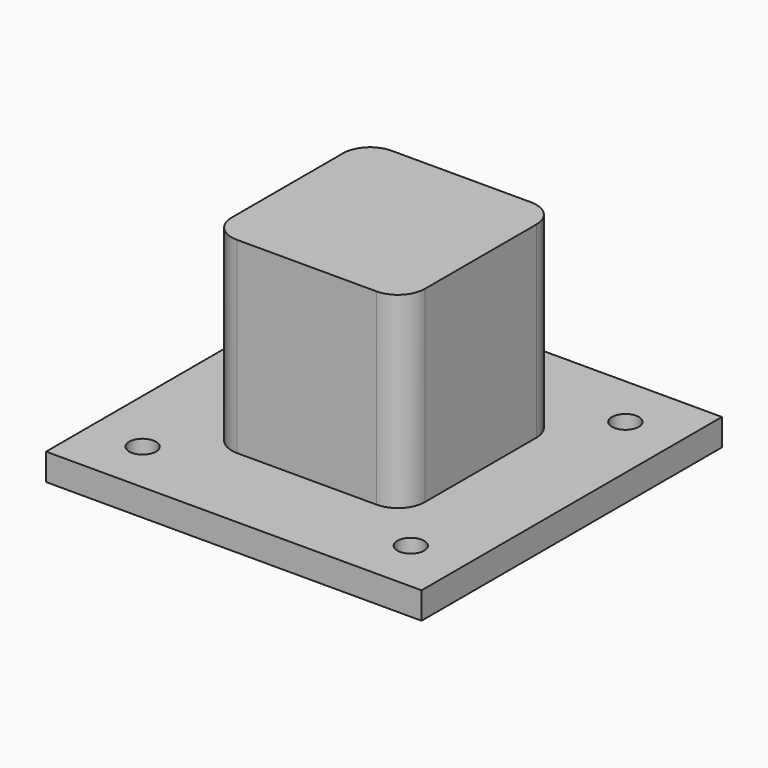
from build123d import *

# Parameters (mm, degrees)
F0_W     = 70
F0_H     = 70
F1_DEPTH = 5
F2_D     = 5
F3_W     = 36
F3_H     = 36
F4_DEPTH = 35
F5_R     = 5


# Not quite as in the source:
# - a feature names something its author has since deleted; it is built from what else it names


with BuildPart() as f1:
    # F0 (on Top) → F1 (new body)
    with BuildSketch(Plane.XY):
        Rectangle(F0_W, F0_H)
    extrude(amount=F1_DEPTH)

    # F2 (through all)
    with Locations(Plane(origin=(0, 0, 0), x_dir=(1, 0, 0), z_dir=(0, 0, -1))):
        with Locations((-25, -25), (25, -25), (25, 25), (-25, 25)):
            Hole(F2_D / 2)

    # F3 (on face) → F4 (join)
    with BuildSketch(Plane.XY.offset(5)):
        Rectangle(F3_W, F3_H)
    extrude(amount=F4_DEPTH)

    # F5
    f5_edges = [f1.edges().sort_by_distance(p)[0] for p in [
        (-18, 18, 22.5),
        (-18, -18, 22.5),
        (18, -18, 22.5),
        (18, 18, 22.5),
    ]]
    fillet(f5_edges, radius=F5_R)


solid = f1.part
